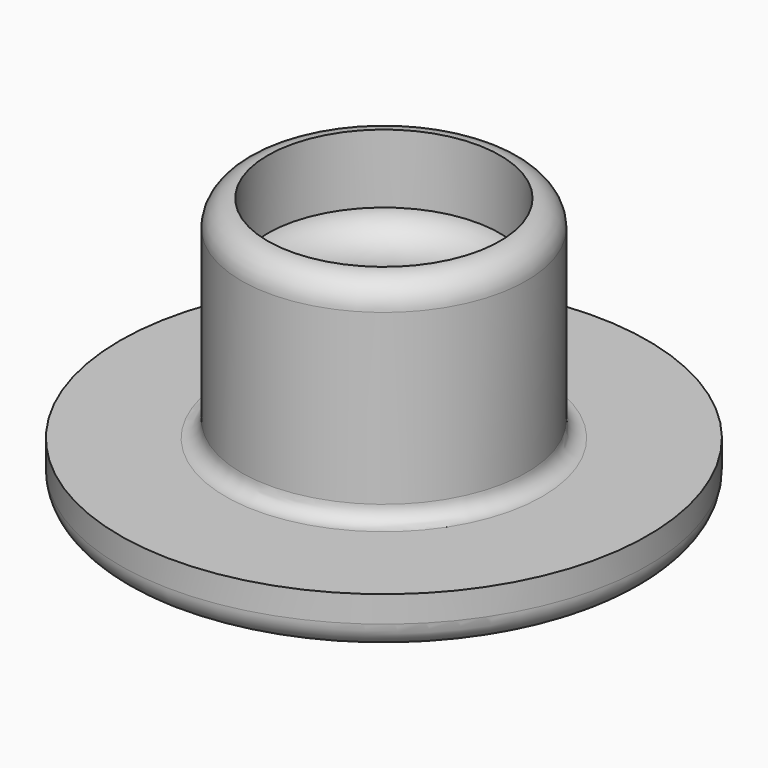
from build123d import *

# Parameters (mm, degrees)
F0_W = 2.2
F0_H = 0.3
F2_R = 0.49999
F3_R = 0.3


# Not quite as in the source:
# - a fillet or chamfer is up to 0.001 mm smaller than in the source, because OpenCascade refuses the exact size


with BuildPart() as f1:
    # F0 (on Front) → F1 (revolve)
    with BuildSketch(Plane.XZ):
        Polygon((-2.7, 1), (-5, 1), (-5, 0), (0, 0), (0, 1), (-2.2, 1), align=None)
        Polygon((-2.7, 5), (-2.7, 1), (-2.2, 1), (-2.2, 1.3), (-2.2, 2.4), (-2.2, 3.7), (-2.2, 5), align=None)
        with BuildLine():
            Line((-2.2, 3.7), (-2.2, 2.4))
            ThreePointArc((-2.2, 2.4), (-1.55, 3.05), (-2.2, 3.7))
        make_face()
        with Locations((-1.1, 1.15)):
            Rectangle(F0_W, F0_H)
    revolve(axis=Axis((0, 0, 0.5), (0, 0, -1)))

    # F2 (radius 0.5 in the source; OpenCascade refuses exactly that, so slightly less here)
    f2_edges = [f1.edges().sort_by_distance(p)[0] for p in [
        (2.7, 0, 5),
        (5, 0, 0),
    ]]
    fillet(f2_edges, radius=F2_R)

    # F3
    f3_edges = [f1.edges().sort_by_distance(p)[0] for p in [
        (2.7, 0, 1),
    ]]
    fillet(f3_edges, radius=F3_R)


solid = f1.part
